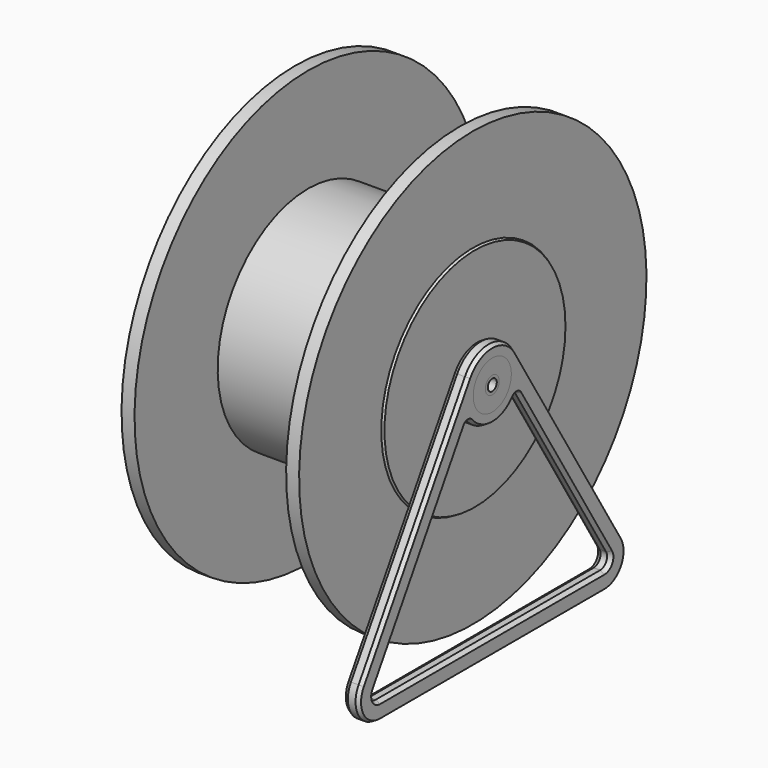
from build123d import *

# Parameters (mm, degrees)
F3_START    = 2
F2_R        = 11
F2_R_2      = 4
F3_DEPTH    = 7
F4_R        = 50.25
F4_R_2      = 2.5
F5_DEPTH    = 6
F5_TAPER    = 1
F6_R        = 53.25
F7_DEPTH    = 1
F8_R        = 4
F8_R_2      = 2.6
F9_DEPTH    = 7
F10_R       = 11
F11_DEPTH   = 7
F13_SIZE2   = 1.1547005384
F13_SIZE    = 2
F14_SIZE2   = 1.7320508076
F14_SIZE    = 1
F14_2_SIZE2 = 1.7320508076
F14_2_SIZE  = 1


# Not quite as in the source:
# - a fillet or chamfer that OpenCascade refuses, or shapes differently, is made with other operations: its cross-section is extruded or revolved along the edge and cut away or added


with BuildPart() as f1:
    # F0 (on Front) → F1 (revolve)
    with BuildSketch(Plane.XZ):
        Polygon((-41, 100.25), (-41, 50.25), (41, 50.25), (41, 100.25), (35, 100.25), (35, 52.25), (-35, 52.25), (-35, 100.25), align=None)
    revolve(axis=Axis((-0.494361277, 0, 0), (1, 0, 0)))


with BuildPart() as f3:
    # F2 (on face) → F3 (new body)
    with BuildSketch(Plane.YZ.offset(41).offset(F3_START)):
        Circle(F2_R)
        Circle(F2_R_2, mode=Mode.SUBTRACT)
    extrude(amount=F3_DEPTH)


with BuildPart() as f5:
    # F4 (on face) → F5 (new body)
    with BuildSketch(Plane.YZ.offset(41)):
        Circle(F4_R)
        Circle(F4_R_2, mode=Mode.SUBTRACT)
    extrude(amount=-F5_DEPTH, taper=F5_TAPER)

    # F6 (on face) → F7 (join)
    with BuildSketch(Plane.YZ.offset(41)):
        Circle(F6_R)
    extrude(amount=F7_DEPTH)

    # F12: chamfer of 1 x 1.7320508076 on 1 edges, made by hand

    # F12_s1 → F12_t2 (revolve, cut)
    with BuildSketch(Plane.XY):
        Polygon((40.2679491924, 53.25), (42, 52.25), (42, 53.25), align=None)
    revolve(axis=Axis((42, 0, 0), (1, 0, 0)), mode=Mode.SUBTRACT)


with BuildPart() as f9:
    # F8 (on face) → F9 (new body, through all)
    with BuildSketch(Plane.YZ.offset(50)):
        Circle(F8_R)
        Circle(F8_R_2, mode=Mode.SUBTRACT)
    extrude(amount=-F9_DEPTH)


with BuildPart() as f11:
    # F10 (on face) → F11 (new body, through all)
    with BuildSketch(Plane.YZ.offset(50)):
        with BuildLine():
            Line((-13.6505324657, 8.3464341728), (-75, -91.9901743704))
            ThreePointArc((-75, -91.9901743704), (-75.2291419603, -104.1186494377), (-64.7621006507, -110.25))
            Line((-64.7621006507, -110.25), (64.7621006507, -110.25))
            ThreePointArc((64.7621006507, -110.25), (75.2291419603, -104.1186494377), (75, -91.9901743704))
            Line((75, -91.9901743704), (13.6505324657, 8.3464341728))
            ThreePointArc((13.6505324657, 8.3464341728), (0, 16), (-13.6505324657, 8.3464341728))
        make_face()
        with BuildLine():
            ThreePointArc((-64.7621006507, -102.25), (-68.2511144206, -100.2062164792), (-68.1747337671, -96.1633914568))
            Line((-68.1747337671, -96.1633914568), (-15.6779965364, -10.3053590236))
            ThreePointArc((-15.6779965364, -10.3053590236), (-14.1049679318, -9.3531096574), (-12.4192710917, -10.0877007068))
            ThreePointArc((-12.4192710917, -10.0877007068), (0, -16), (12.4192710917, -10.0877007068))
            ThreePointArc((12.4192710917, -10.0877007068), (14.1049679318, -9.3531096574), (15.6779965364, -10.3053590236))
            Line((15.6779965364, -10.3053590236), (68.1747337671, -96.1633914568))
            ThreePointArc((68.1747337671, -96.1633914568), (68.2511144206, -100.2062164792), (64.7621006507, -102.25))
            Line((64.7621006507, -102.25), (-64.7621006507, -102.25))
        make_face(mode=Mode.SUBTRACT)
        Circle(F10_R, mode=Mode.SUBTRACT)
    extrude(amount=-F11_DEPTH)

    # F13
    f13_edges = [f11.edges().sort_by_distance(p)[0] for p in [
        (50, 0, -102.25),
        (43, 0, -102.25),
    ]]
    f13_side = f11.faces().sort_by_distance((46.5, 0, -102.25))[0]
    chamfer(f13_edges, length=F13_SIZE, length2=F13_SIZE2, reference=f13_side)

    # F14
    f14_edges = [f11.edges().sort_by_distance(p)[0] for p in [
        (50, 0, -110.25),
    ]]
    f14_side = f11.faces().sort_by_distance((50, 0, -105.392381))[0]
    chamfer(f14_edges, length=F14_SIZE, length2=F14_SIZE2, reference=f14_side)

    # F14#2
    f14_2_edges = [f11.edges().sort_by_distance(p)[0] for p in [
        (43, 0, -110.25),
    ]]
    f14_2_side = f11.faces().sort_by_distance((43, 0, -105.392381))[0]
    chamfer(f14_2_edges, length=F14_2_SIZE, length2=F14_2_SIZE2, reference=f14_2_side)


solid = Compound([f1.part, f3.part, f5.part, f9.part, f11.part])
